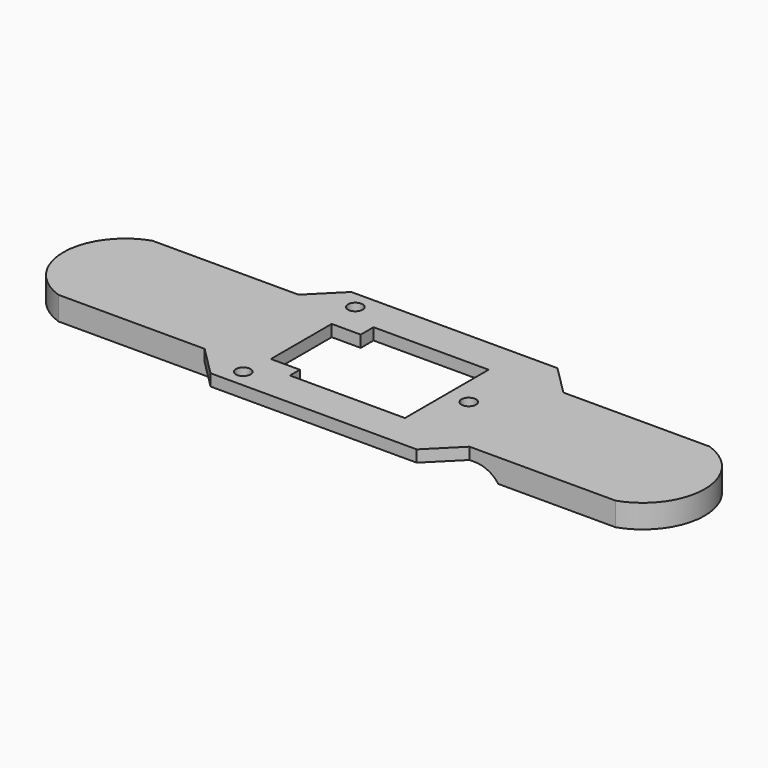
from build123d import *

# Parameters (mm, degrees)
F0_W         = 35
F0_H         = 30
F0_R         = 1.25
F1_DEPTH     = 2
F2_W         = 20
F2_H         = 20
F2_W_2       = 30
F2_W_3       = 10
F3_DEPTH     = 4
F4_T4_DEPTH  = 2
F4_T9_DEPTH  = 2
F4_T14_DEPTH = 2
F4_T19_DEPTH = 2
F6_SIZE      = 5.08
F7_SIZE      = 5.08
F9_DEPTH     = 2
F10_T1_DEPTH = 20


# Not quite as in the source:
# - a fillet or chamfer that OpenCascade refuses, or shapes differently, is made with other operations: its cross-section is extruded or revolved along the edge and cut away or added
# - a feature of the source that left no trace in its solid (it failed there, or was rolled back) is left out


with BuildPart() as f1:
    # F0 (on Top) → F1 (new body)
    with BuildSketch(Plane.XY):
        Rectangle(F0_W, F0_H)
        with Locations((-14.45, -11.95)):
            Circle(F0_R, mode=Mode.SUBTRACT)
        Polygon((-8.9161582291, 8.9178942144), (8.9161582291, 8.9178942144), (10.7079278678, 8.9178942144), (10.7079250291, -8.9178942144), (8.9161582291, -8.9178942144), (-8.9161582291, -8.9178942144), (-8.9161582291, -6.7814155482), (-13.8649037108, -6.7814155482), (-13.8649037108, 6.1875791289), (-8.9161582291, 6.1875791289), align=None, mode=Mode.SUBTRACT)
        with Locations((-14.45, 11.95)):
            Circle(F0_R, mode=Mode.SUBTRACT)
        with Locations((14.45, 0)):
            Circle(F0_R, mode=Mode.SUBTRACT)
    extrude(amount=F1_DEPTH)

    # F2 (on face) → F3 (join)
    with BuildSketch(Plane.XY.offset(2)):
        with BuildLine():
            Line((47.5, 10), (47.5, -10))
            ThreePointArc((47.5, -10), (54.6755987692, 0), (47.5, 10))
        make_face()
        with BuildLine():
            ThreePointArc((-47.5, 10), (-54.6755833881, 0), (-47.5, -10))
            Line((-47.5, -10), (-47.5, 10))
        make_face()
        with Locations((37.5, 0)):
            Rectangle(F2_W, F2_H)
        with Locations((-32.5, 0)):
            Rectangle(F2_W_2, F2_H)
        with Locations((22.5, 0)):
            Rectangle(F2_W_3, F2_H)
    extrude(amount=-F3_DEPTH)

    # F4: chamfer of 5.08 on 4 edges, made by hand


with BuildPart() as f4_tool2:
    # F4_s3 → F4_t4 (new body)
    with BuildSketch(Plane.XY.offset(2)):
        Polygon((-17.5, 15.08), (-22.58, 10), (-17.5, 10), align=None)
    extrude(amount=-F4_T4_DEPTH)

    split(bisect_by=Plane.XZ.offset(-15), keep=Keep.TOP)


with BuildPart() as f1_1:
    add(f1.part)

    # F4_t1: union F4_tool2
    add(f4_tool2.part)


with BuildPart() as f4_tool7:
    # F4_s8 → F4_t9 (new body)
    with BuildSketch(Plane.XY.offset(2)):
        Polygon((17.5, -15.08), (22.58, -10), (17.5, -10), align=None)
    extrude(amount=-F4_T9_DEPTH)

    split(bisect_by=Plane.XZ.offset(15), keep=Keep.BOTTOM)


with BuildPart() as f1_2:
    add(f1_1.part)

    # F4_t6: union F4_tool7
    add(f4_tool7.part)


with BuildPart() as f4_tool12:
    # F4_s13 → F4_t14 (new body)
    with BuildSketch(Plane.XY.offset(2)):
        Polygon((17.5, 15.08), (22.58, 10), (17.5, 10), align=None)
    extrude(amount=-F4_T14_DEPTH)

    split(bisect_by=Plane.XZ.offset(-15), keep=Keep.TOP)


with BuildPart() as f1_3:
    add(f1_2.part)

    # F4_t11: union F4_tool12
    add(f4_tool12.part)


with BuildPart() as f4_tool17:
    # F4_s18 → F4_t19 (new body)
    with BuildSketch(Plane.XY.offset(2)):
        Polygon((-17.5, -15.08), (-22.58, -10), (-17.5, -10), align=None)
    extrude(amount=-F4_T19_DEPTH)

    split(bisect_by=Plane.XZ.offset(15), keep=Keep.BOTTOM)


with BuildPart() as f1_4:
    add(f1_3.part)

    # F4_t16: union F4_tool17
    add(f4_tool17.part)

    # F6
    f6_edges = [f1_4.edges().sort_by_distance(p)[0] for p in [
        (17.5, -10, -1),
    ]]
    chamfer(f6_edges, length=F6_SIZE)

    # F7
    f7_edges = [f1_4.edges().sort_by_distance(p)[0] for p in [
        (17.5, 10, -1),
    ]]
    chamfer(f7_edges, length=F7_SIZE)

    # F8 (on face) → F9 (cut)
    with BuildSketch(Plane(origin=(0, 0, -2), x_dir=(1, 0, 0), z_dir=(0, 0, -1))):
        Polygon((27.5, -10), (27.5, 10), (22.58, 10), (17.5, 4.92), (17.5, -4.92), (22.58, -10), align=None)
    extrude(amount=-F9_DEPTH, mode=Mode.SUBTRACT)

    # F10: fillet of radius 5.08 on 1 edges, made by hand

    # F10_s2 → F10_t1 (join)
    with BuildSketch(Plane.XZ.offset(-10)):
        with BuildLine():
            ThreePointArc((27.5, -2), (25.7140835586, -0.5273743839), (23.4601980247, 0))
            Line((23.4601980247, 0), (27.5, 0))
            Line((27.5, 0), (27.5, -2))
        make_face()
    extrude(amount=F10_T1_DEPTH)


solid = f1_4.part
